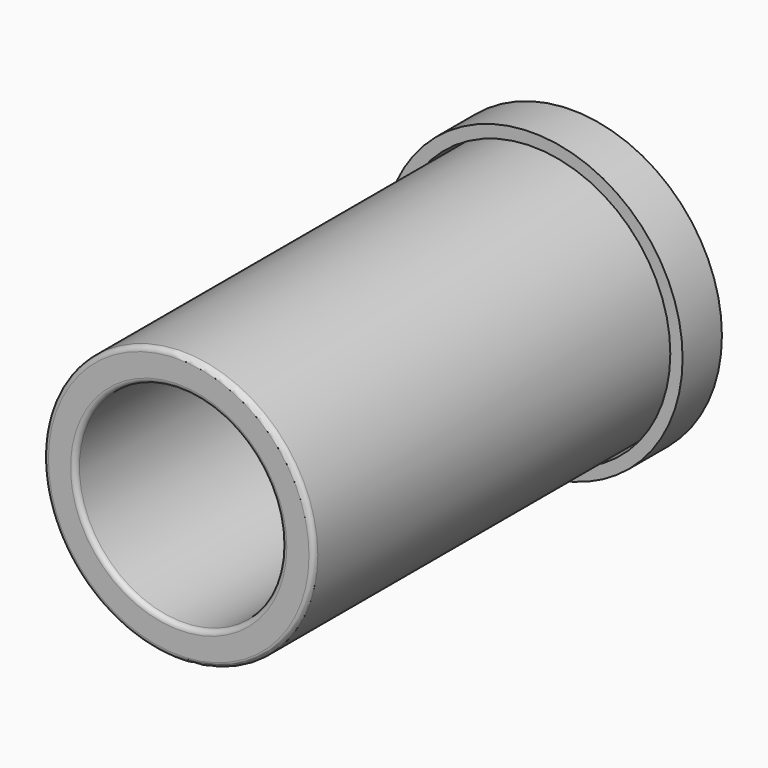
from build123d import *

# Parameters (mm, degrees)
F0_R     = 15.25
F0_R_2   = 14
F1_DEPTH = 5
F0_R_3   = 13.75
F0_R_4   = 10.5
F3_DEPTH = 50
F4_R     = 0.5
F5_R     = 0.5


# Not quite as in the source:
# - the program builds the solid bodies; features that only make, move or delete a surface that nothing else refers to are left out


with BuildPart() as f1:
    # F0 (on Front) → F1 (new body)
    with BuildSketch(Plane.XZ):
        Circle(F0_R)
        Circle(F0_R_2, mode=Mode.SUBTRACT)
    extrude(amount=F1_DEPTH)


with BuildPart() as f3:
    # F0 (on Front) → F3 (new body)
    with BuildSketch(Plane.XZ):
        Circle(F0_R_3)
        Circle(F0_R_4, mode=Mode.SUBTRACT)
    extrude(amount=F3_DEPTH)

    # F4
    f4_edges = [f3.edges().sort_by_distance(p)[0] for p in [
        (-13.75, -50, 0),
        (-10.5, -50, 0),
    ]]
    fillet(f4_edges, radius=F4_R)

    # F5
    f5_edges = [f3.edges().sort_by_distance(p)[0] for p in [
        (-10.5, 0, 0),
    ]]
    fillet(f5_edges, radius=F5_R)


solid = Compound([f1.part, f3.part])
